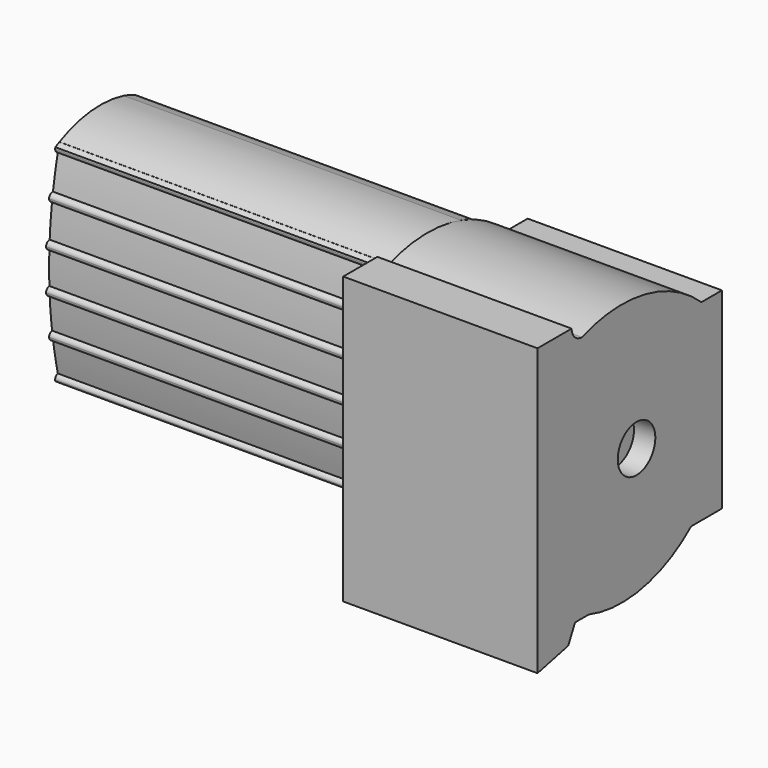
from build123d import *

# Parameters (mm, degrees)
F1_DEPTH = 45.5
F2_R     = 5.5
F3_DEPTH = 5
F5_DEPTH = 79
F7_DEPTH = 4


# Not quite as in the source:
# - ends of sketch curves that miss each other by under 0.0002 mm in the source are joined


with BuildPart() as f1:
    # F0 (on Right) → F1 (new body)
    with BuildSketch(Plane.YZ):
        with BuildLine():
            Line((-9, 0), (0, 0))
            Line((0, 0), (0, 45))
            Line((0, 45), (-6, 45))
            ThreePointArc((-6, 45), (-22.5330315813, 53.3348420934), (-41, 52))
            ThreePointArc((-41, 52), (-43.1213203436, 52.8786796564), (-44, 55))
            Line((-44, 55), (-54, 55))
            Line((-54, 55), (-54, -12.0034376159))
            Line((-54, -12.0034376159), (-45, -10))
            Line((-45, -10), (-43, -6))
            Line((-43, -6), (-39, -6))
            ThreePointArc((-39, -6), (-23.216376947, -6.9181152652), (-9, 0))
        make_face()
    extrude(amount=-F1_DEPTH)

    # F2 (on face) → F3 (cut)
    with BuildSketch(Plane.YZ):
        with Locations((-25, 22.5448962301)):
            Circle(F2_R)
    extrude(amount=-F3_DEPTH, mode=Mode.SUBTRACT)


with BuildPart() as f5:
    # F4 (on face) → F5 (new body)
    with BuildSketch(Plane(origin=(-45.5, 0, 0), x_dir=(0, -1, 0), z_dir=(-1, 0, 0))):
        with BuildLine():
            ThreePointArc((39.5914929211, 49.738612026), (39.5745273011, 49.9220334198), (39.5242061057, 50.0992310984))
            ThreePointArc((39.5242061057, 50.0992310984), (38.9457342247, 50.4057503771), (38.3601298002, 50.698412714))
            ThreePointArc((38.3601298002, 50.698412714), (38.5929522401, 49.7324279994), (38.8164939134, 48.7642534916))
            ThreePointArc((38.8164939134, 48.7642534916), (39.3741170302, 49.1161174446), (39.5914929211, 49.738612026))
        make_face()
    extrude(amount=F5_DEPTH)


with BuildPart() as f5b:
    # F4 (on face) → F5, piece 2 (new body)
    with BuildSketch(Plane(origin=(-45.5, 0, 0), x_dir=(0, -1, 0), z_dir=(-1, 0, 0))):
        with BuildLine():
            ThreePointArc((38.3601298002, 1.2110405874), (38.9450870807, 1.5033698326), (39.5229280333, 1.8095254158))
            ThreePointArc((39.5229280333, 1.8095254158), (39.5753429364, 1.9901153498), (39.5930229595, 2.1773250267))
            ThreePointArc((39.5930229595, 2.1773250267), (39.3756270427, 2.7998447846), (38.8179612614, 3.1516980355))
            ThreePointArc((38.8179612614, 3.1516980355), (38.5937171125, 2.1802672122), (38.3601298002, 1.2110405874))
        make_face()
    extrude(amount=F5_DEPTH)


with BuildPart() as f5c:
    # F4 (on face) → F5, piece 3 (new body)
    with BuildSketch(Plane(origin=(-45.5, 0, 0), x_dir=(0, -1, 0), z_dir=(-1, 0, 0))):
        with BuildLine():
            ThreePointArc((38.8164939134, 48.7642534916), (37.6200137516, 49.5014871154), (38.342280913, 50.7070609792))
            ThreePointArc((38.342280913, 50.7070609792), (29.091484933, 53.3187486346), (19.5069737394, 52.5871176813))
            ThreePointArc((19.5069737394, 52.5871176813), (17.8887038243, 52.065983046), (16.297847496, 51.4663540199))
            ThreePointArc((16.297847496, 51.4663540199), (9.360167175, 25.8933628751), (16.3601298002, 0.3373497358))
            ThreePointArc((16.3601298002, 0.3373497358), (27.4466468085, -1.5238009807), (38.3515991148, 1.2069052581))
            ThreePointArc((38.3515991148, 1.2069052581), (37.6205916355, 2.4105144775), (38.8179612614, 3.1516980355))
            ThreePointArc((38.8179612614, 3.1516980355), (39.5938697508, 6.9115298603), (40.2298639805, 10.6975410429))
            ThreePointArc((40.2298639805, 10.6975410429), (39.3819781674, 11.8251188452), (40.5054484043, 12.678439816))
            ThreePointArc((40.5054484043, 12.678439816), (40.9213150894, 16.432192603), (41.2000084443, 20.1986146585))
            ThreePointArc((41.2000084443, 20.1986146585), (40.2518346275, 21.2432717627), (41.2919008449, 22.1964791461))
            ThreePointArc((41.2919008449, 22.1964791461), (41.3601297494, 25.9579719584), (41.291665052, 29.7194604864))
            ThreePointArc((41.291665052, 29.7194604864), (40.2515390839, 30.6726026702), (41.1996474134, 31.7173192096))
            ThreePointArc((41.1996474134, 31.7173192096), (40.9207153981, 35.4837514741), (40.5046088311, 39.2375056479))
            ThreePointArc((40.5046088311, 39.2375056479), (39.3810846469, 40.0907555877), (40.2288991693, 41.2183869938))
            ThreePointArc((40.2288991693, 41.2183869938), (39.5926549425, 45.0044147778), (38.8164939134, 48.7642534916))
        make_face()
    extrude(amount=F5_DEPTH)

    # F6 (on face) → F7 (cut)
    with BuildSketch(Plane(origin=(-124.5, 0, 0), x_dir=(0, -1, 0), z_dir=(-1, 0, 0))):
        with BuildLine():
            ThreePointArc((26.1499717328, 21.9602512675), (22.519565713, 24.8366624789), (24.0387774872, 29.212229289))
            Line((24.0387774872, 29.212229289), (9.6729229343, 31.5597305505))
            ThreePointArc((9.6729229343, 31.5597305505), (9.3706290349, 26.98316608), (9.4858426199, 22.3980761372))
            Line((9.4858426199, 22.3980761372), (26.1499717328, 21.9602512675))
        make_face()
        with BuildLine():
            ThreePointArc((26.3601298002, 21.9547266507), (29.188556925, 23.1262995259), (30.3601298002, 25.9547266507))
            ThreePointArc((30.3601298002, 25.9547266507), (28.1924221824, 29.510384765), (24.0387774872, 29.212229289))
            ThreePointArc((24.0387774872, 29.212229289), (22.519565713, 24.8366624789), (26.1499717328, 21.9602512675))
            Line((26.1499717328, 21.9602512675), (26.3601298002, 21.9547266507))
        make_face()
    extrude(amount=-F7_DEPTH, mode=Mode.SUBTRACT)


with BuildPart() as f5d:
    # F4 (on face) → F5, piece 4 (new body)
    with BuildSketch(Plane(origin=(-45.5, 0, 0), x_dir=(0, -1, 0), z_dir=(-1, 0, 0))):
        with BuildLine():
            ThreePointArc((41.3715368681, 40.228612026), (41.026274335, 40.9844683942), (40.2288991693, 41.2183869938))
            ThreePointArc((40.2288991693, 41.2183869938), (40.3715368681, 40.228612026), (40.5046088311, 39.2375056479))
            ThreePointArc((40.5046088311, 39.2375056479), (41.1242227133, 39.5702321824), (41.3715368681, 40.228612026))
        make_face()
    extrude(amount=F5_DEPTH)


with BuildPart() as f5e:
    # F4 (on face) → F5, piece 5 (new body)
    with BuildSketch(Plane(origin=(-45.5, 0, 0), x_dir=(0, -1, 0), z_dir=(-1, 0, 0))):
        with BuildLine():
            ThreePointArc((40.5054484043, 12.678439816), (40.3724391024, 11.6873250267), (40.2298639805, 10.6975410429))
            ThreePointArc((40.2298639805, 10.6975410429), (41.0272004628, 10.9314893561), (41.3724391024, 11.6873250267))
            ThreePointArc((41.3724391024, 11.6873250267), (41.1251041347, 12.3457286635), (40.5054484043, 12.678439816))
        make_face()
    extrude(amount=F5_DEPTH)


with BuildPart() as f5f:
    # F4 (on face) → F5, piece 6 (new body)
    with BuildSketch(Plane(origin=(-45.5, 0, 0), x_dir=(0, -1, 0), z_dir=(-1, 0, 0))):
        with BuildLine():
            ThreePointArc((42.2504800927, 30.718612026), (41.9393804196, 31.443468108), (41.1996474134, 31.7173192096))
            ThreePointArc((41.1996474134, 31.7173192096), (41.2504800927, 30.718612026), (41.291665052, 29.7194604864))
            ThreePointArc((41.291665052, 29.7194604864), (41.9720010416, 30.0262194203), (42.2504800927, 30.718612026))
        make_face()
    extrude(amount=F5_DEPTH)


with BuildPart() as f5g:
    # F4 (on face) → F5, piece 7 (new body)
    with BuildSketch(Plane(origin=(-45.5, 0, 0), x_dir=(0, -1, 0), z_dir=(-1, 0, 0))):
        with BuildLine():
            ThreePointArc((41.2919008449, 22.1964791461), (41.2507785185, 21.1973250267), (41.2000084443, 20.1986146585))
            ThreePointArc((41.2000084443, 20.1986146585), (41.9397015642, 20.4724905372), (42.2507785185, 21.1973250267))
            ThreePointArc((42.2507785185, 21.1973250267), (41.9722777654, 21.8897402466), (41.2919008449, 22.1964791461))
        make_face()
    extrude(amount=F5_DEPTH)


solid = Compound([f1.part, f5.part, f5b.part, f5c.part, f5d.part, f5e.part, f5f.part, f5g.part])
